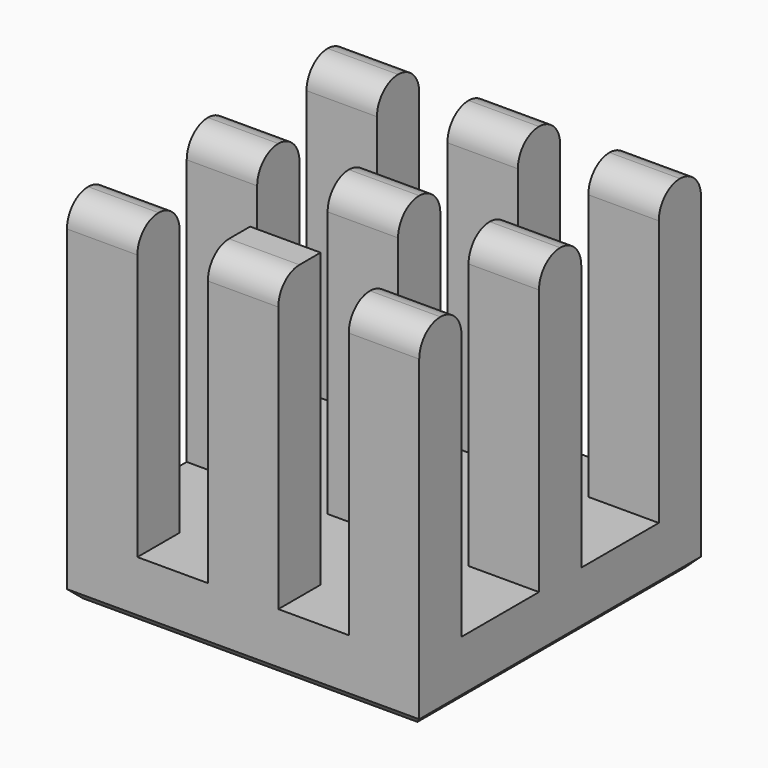
from build123d import *

# Parameters (mm, degrees)
F0_W     = 10
F0_H     = 10
F1_DEPTH = 1.7
F2_SIZE  = 0.25
F3_W     = 2
F3_H     = 1.5
F4_DEPTH = 8.3
F5_R     = 0.74999


# Not quite as in the source:
# - a fillet or chamfer is up to 0.001 mm smaller than in the source, because OpenCascade refuses the exact size


with BuildPart() as f1:
    # F0 (on Top) → F1 (new body)
    with BuildSketch(Plane.XY):
        with Locations((5, 5)):
            Rectangle(F0_W, F0_H)
    extrude(amount=F1_DEPTH)

    # F2
    f2_edges = [f1.edges().sort_by_distance(p)[0] for p in [
        (5, 0, 0),
        (0, 5, 0),
        (10, 5, 0),
        (5, 10, 0),
    ]]
    chamfer(f2_edges, length=F2_SIZE)

    # F3 (on face) → F4 (join)
    with BuildSketch(Plane.XY.offset(1.7)):
        with Locations((1, 9.25)):
            Rectangle(F3_W, F3_H)
        with Locations((9, 9.25)):
            Rectangle(F3_W, F3_H)
        with Locations((1, 0.75)):
            Rectangle(F3_W, F3_H)
        with Locations((9, 0.75)):
            Rectangle(F3_W, F3_H)
        with Locations((1, 5)):
            Rectangle(F3_W, F3_H)
        with Locations((5, 9.25)):
            Rectangle(F3_W, F3_H)
        with Locations((9, 5)):
            Rectangle(F3_W, F3_H)
        with Locations((5, 5)):
            Rectangle(F3_W, F3_H)
        with Locations((5, 0.75)):
            Rectangle(F3_W, F3_H)
    extrude(amount=F4_DEPTH)

    # F5 (radius 0.75 in the source; OpenCascade refuses exactly that, so slightly less here)
    f5_edges = [f1.edges().sort_by_distance(p)[0] for p in [
        (1, 0, 10),
        (1, 1.5, 10),
        (5, 0, 10),
        (9, 0, 10),
        (9, 1.5, 10),
        (9, 4.25, 10),
        (9, 5.75, 10),
        (5, 4.25, 10),
        (5, 5.75, 10),
        (1, 4.25, 10),
        (1, 5.75, 10),
        (1, 8.5, 10),
        (1, 10, 10),
        (5, 8.5, 10),
        (5, 10, 10),
        (9, 8.5, 10),
        (9, 10, 10),
    ]]
    fillet(f5_edges, radius=F5_R)


solid = f1.part
